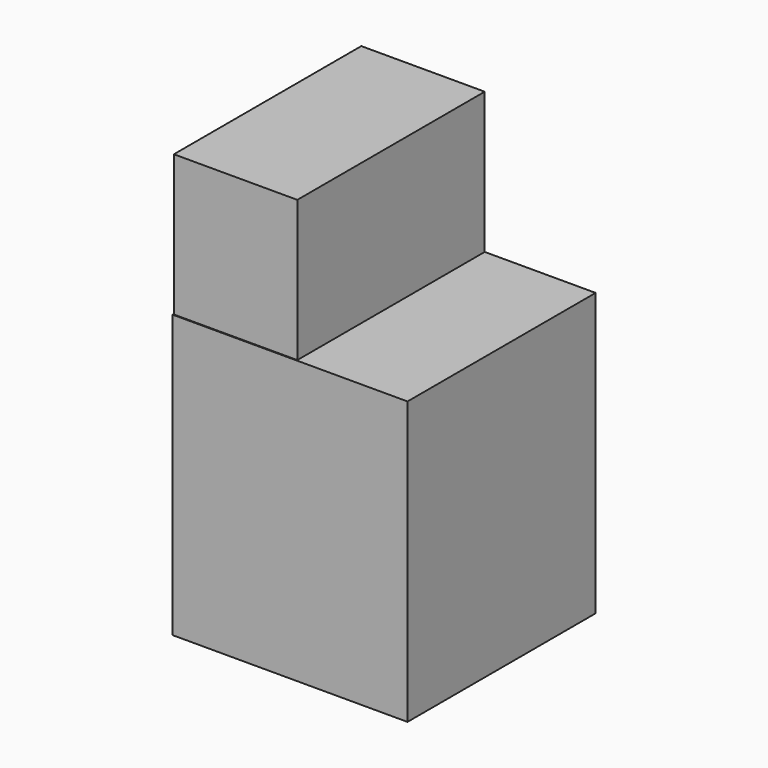
from build123d import *

# Parameters (mm, degrees)
F0_W     = 10000
F0_H     = 10000
F1_DEPTH = 12000
F3_W     = 5250
F3_H     = 9963.928271085
F5_DEPTH = 6000


# Not quite as in the source:
# - a feature of the source that left no trace in its solid (it failed there, or was rolled back) is left out


with BuildPart() as f1:
    # F0 (on Top) → F1 (new body)
    with BuildSketch(Plane.XY):
        with Locations((4965.7781012356, 4963.928271085)):
            Rectangle(F0_W, F0_H)
    extrude(amount=F1_DEPTH)

    # F3 (on face) → F5 (join)
    with BuildSketch(Plane.XY.offset(12000)):
        with Locations((2625, 4981.9641355425)):
            Rectangle(F3_W, F3_H)
    extrude(amount=F5_DEPTH)


solid = f1.part
